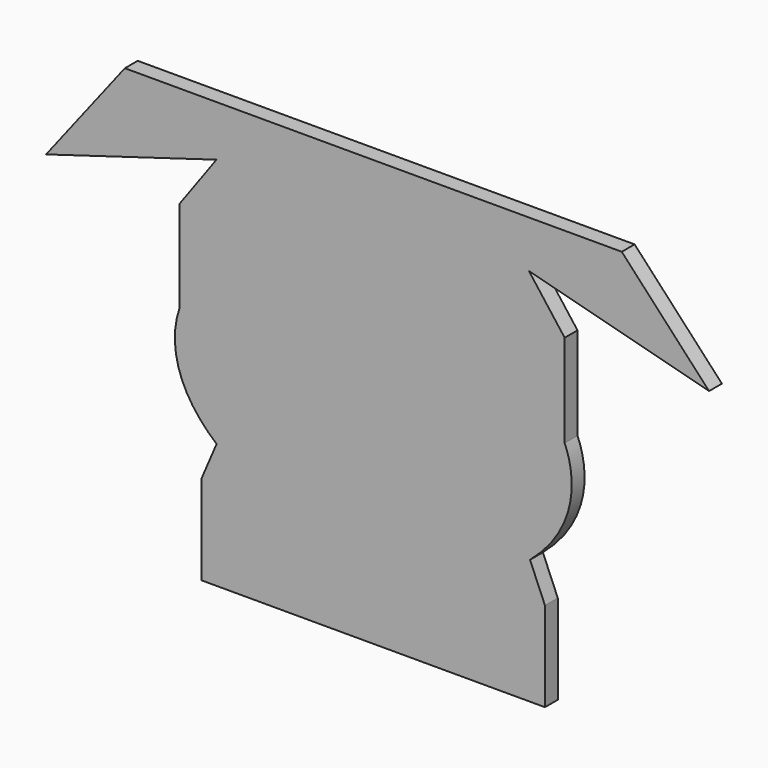
from build123d import *

# Parameters (mm, degrees)
F0_W     = 22.0716209825
F0_H     = 11.3639943302
F0_W_2   = 22.1128826787
F1_DEPTH = 3.175


with BuildPart() as f1:
    # F0 (on Front) → F1 (new body)
    with BuildSketch(Plane.XZ):
        with BuildLine():
            add(Edge.make_bspline(
                [(0, 77.2495130793), (-13.2024395854, 77.2495130793), (-23.7188442589, 72.0280801734)],
                knots=[1.5707963268, 1.5707963268, 1.5707963268, 2.2200254143, 2.2200254143, 2.2200254143], degree=2, weights=[1, 0.9477737356, 1]))
            ThreePointArc((0, 77.2495130793), (-14.9655593265, 88.7487135304), (-23.7188442589, 72.0280801734))
        make_face()
        with BuildLine():
            add(Edge.make_bspline(
                [(37.8281886895, 58.3899668587), (34.3045126324, 66.7722575902), (23.7188442589, 72.0280801734)],
                knots=[0.2683589556, 0.2683589556, 0.2683589556, 0.9215672393, 0.9215672393, 0.9215672393], degree=2, weights=[1, 0.9471372908, 1]))
            add(Edge.make_bspline(
                [(23.7188442589, 72.0280801734), (13.2024395854, 77.2495130793), (0, 77.2495130793)],
                knots=[0.9215672393, 0.9215672393, 0.9215672393, 1.5707963268, 1.5707963268, 1.5707963268], degree=2, weights=[1, 0.9477737356, 1]))
            add(Edge.make_bspline(
                [(0, 77.2495130793), (-13.2024395854, 77.2495130793), (-23.7188442589, 72.0280801734)],
                knots=[1.5707963268, 1.5707963268, 1.5707963268, 2.2200254143, 2.2200254143, 2.2200254143], degree=2, weights=[1, 0.9477737356, 1]))
            add(Edge.make_bspline(
                [(-23.7188442589, 72.0280801734), (-35.179956424, 66.3375965856), (-38.2993388492, 57.1490477352)],
                knots=[2.2200254143, 2.2200254143, 2.2200254143, 2.9230595545, 2.9230595545, 2.9230595545], degree=2, weights=[1, 0.9388514321, 1]))
            add(Edge.make_bspline(
                [(-38.2993388492, 57.1490477352), (-42.2983339169, 45.3694848208), (-30.9822451126, 35.8404089541)],
                knots=[2.9230595545, 2.9230595545, 2.9230595545, 3.8020524721, 3.8020524721, 3.8020524721], degree=2, weights=[1, 0.9049660266, 1]))
            Line((-30.9822451126, 35.8404089541), (-33.9723048082, 28.8538616849))
            Line((-33.9723048082, 28.8538616849), (-33.9723048082, 22.5029981736))
            Line((-33.9723048082, 22.5029981736), (-11.8594221295, 22.5029981736))
            Line((-11.8594221295, 22.5029981736), (-11.8594221295, 11.1390038435))
            Line((-11.8594221295, 11.1390038435), (11.8594221295, 11.1390038435))
            Line((11.8594221295, 11.1390038435), (11.8594221295, 22.5029981736))
            Line((11.8594221295, 22.5029981736), (33.931043112, 22.5029981736))
            Line((33.931043112, 22.5029981736), (33.931043112, 28.8538616849))
            Line((33.931043112, 28.8538616849), (30.9822451126, 35.8404089541))
            add(Edge.make_bspline(
                [(30.9822451126, 35.8404089541), (43.0393262584, 45.9934612106), (37.8281886895, 58.3899668587)],
                knots=[5.6227254887, 5.6227254887, 5.6227254887, 6.5515442627, 6.5515442627, 6.5515442627], degree=2, weights=[1, 0.894086254, 1]))
        make_face()
        with BuildLine():
            add(Edge.make_bspline(
                [(23.7188442589, 57.1490477352), (23.7188442589, 89.4658166317), (-16.7717556174, 66.614410199), (-57.2623554937, 43.7630037663), (0, 43.7630037663)],
                knots=[0, 0, 0, 2.3561944902, 2.3561944902, 4.7123889804, 4.7123889804, 4.7123889804], degree=2, weights=[1, 0.3826834324, 1, 0.3826834324, 1]))
            add(Edge.make_bspline(
                [(0, 43.7630037663), (23.7188442589, 43.7630037663), (23.7188442589, 57.1490477352)],
                knots=[4.7123889804, 4.7123889804, 4.7123889804, 6.2831853072, 6.2831853072, 6.2831853072], degree=2, weights=[1, 0.7071067812, 1]))
        make_face(mode=Mode.SUBTRACT)
        with Locations((22.8952326207, 16.8210010086)):
            Rectangle(F0_W, F0_H)
        with BuildLine():
            add(Edge.make_bspline(
                [(23.7188442589, 72.0280801734), (13.2024395854, 77.2495130793), (0, 77.2495130793)],
                knots=[0.9215672393, 0.9215672393, 0.9215672393, 1.5707963268, 1.5707963268, 1.5707963268], degree=2, weights=[1, 0.9477737356, 1]))
            ThreePointArc((23.7188442589, 72.0280801734), (14.8063132284, 88.0253233293), (0, 77.2495130793))
        make_face()
        with BuildLine():
            add(Edge.make_bspline(
                [(0, 43.7630037663), (23.7188442589, 43.7630037663), (23.7188442589, 57.1490477352)],
                knots=[4.7123889804, 4.7123889804, 4.7123889804, 6.2831853072, 6.2831853072, 6.2831853072], degree=2, weights=[1, 0.7071067812, 1]))
            add(Edge.make_bspline(
                [(23.7188442589, 57.1490477352), (23.7188442589, 89.4658166317), (-16.7717556174, 66.614410199), (-57.2623554937, 43.7630037663), (0, 43.7630037663)],
                knots=[0, 0, 0, 2.3561944902, 2.3561944902, 4.7123889804, 4.7123889804, 4.7123889804], degree=2, weights=[1, 0.3826834324, 1, 0.3826834324, 1]))
        make_face()
        with BuildLine():
            ThreePointArc((0, 77.2495130793), (14.8063132284, 88.0253233293), (23.7188442589, 72.0280801734))
            add(Edge.make_bspline(
                [(37.8281886895, 58.3899668587), (34.3045126324, 66.7722575902), (23.7188442589, 72.0280801734)],
                knots=[0.2683589556, 0.2683589556, 0.2683589556, 0.9215672393, 0.9215672393, 0.9215672393], degree=2, weights=[1, 0.9471372908, 1]))
            Line((37.8281886895, 58.3899668587), (37.8281886895, 76.7098173911))
            Line((37.8281886895, 76.7098173911), (30.7735164742, 86.026978908))
            Line((30.7735164742, 86.026978908), (66.3792615504, 76.7098173911))
            Line((66.3792615504, 76.7098173911), (49.1188442589, 95.3441404248))
            Line((49.1188442589, 95.3441404248), (23.7188442589, 95.3441404248))
            Line((23.7188442589, 95.3441404248), (-23.7188442589, 95.3441404248))
            Line((-23.7188442589, 95.3441404248), (-49.1188442589, 95.3441404248))
            Line((-49.1188442589, 95.3441404248), (-64.6933734609, 75.2793942231))
            Line((-64.6933734609, 75.2793942231), (-31.0090915541, 85.311767324))
            Line((-31.0090915541, 85.311767324), (-38.2993388492, 75.2793942231))
            Line((-38.2993388492, 75.2793942231), (-38.2993388492, 57.1490477352))
            add(Edge.make_bspline(
                [(-23.7188442589, 72.0280801734), (-35.179956424, 66.3375965856), (-38.2993388492, 57.1490477352)],
                knots=[2.2200254143, 2.2200254143, 2.2200254143, 2.9230595545, 2.9230595545, 2.9230595545], degree=2, weights=[1, 0.9388514321, 1]))
            ThreePointArc((-23.7188442589, 72.0280801734), (-14.9655593265, 88.7487135304), (0, 77.2495130793))
        make_face()
        with Locations((-22.9158634688, 16.8210010086)):
            Rectangle(F0_W_2, F0_H)
    extrude(amount=-F1_DEPTH)


solid = f1.part
